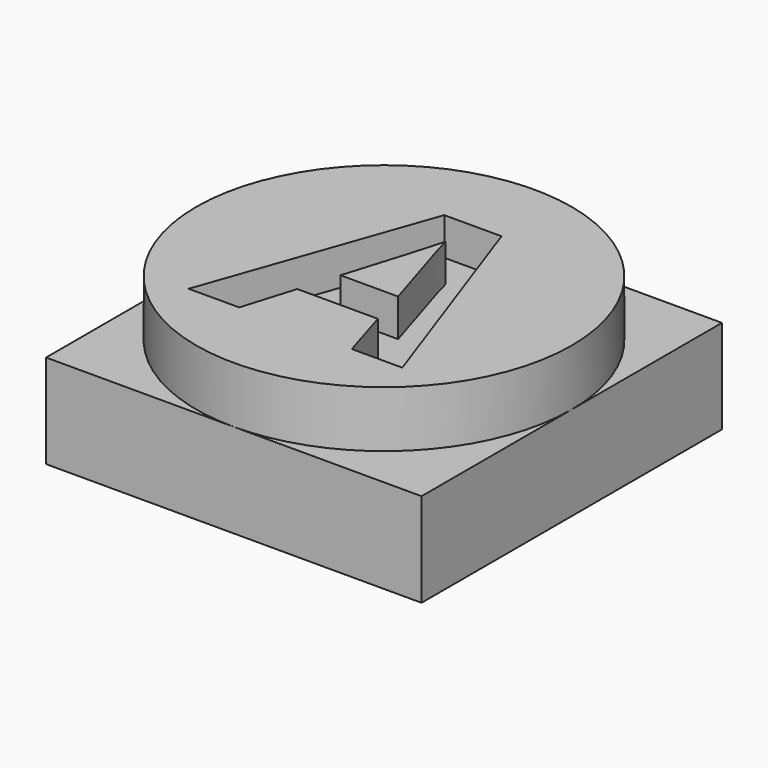
from build123d import *

# Parameters (mm, degrees)
F0_W         = 20
F0_H         = 20
F1_DEPTH     = 5
F2_R         = 10
F3_DEPTH     = 3
F4_TEXT_SIZE = 16.4918847279
F5_DEPTH     = 2


# Not quite as in the source:
# - Text() gives the source's letters only with a copy of the font that has no kerning and outlines rounded to 1/6400 em; it was checked with that copy


with BuildPart() as f1:
    # F0 (on Top) → F1 (new body)
    with BuildSketch(Plane.XY):
        Rectangle(F0_W, F0_H)
    extrude(amount=F1_DEPTH)

    # F2 (on face) → F3 (join)
    with BuildSketch(Plane.XY.offset(5)):
        Circle(F2_R)
    extrude(amount=F3_DEPTH)

    # F4 (on face) → F5 (cut)
    with BuildSketch(Plane.XY.offset(8)):
        with Locations((-5.636760965, -5.9601804242)):
            Text('A', F4_TEXT_SIZE, font='Open Sans', font_style=FontStyle.BOLD, text_align=(TextAlign.LEFT, TextAlign.BOTTOM))
    extrude(amount=-F5_DEPTH, mode=Mode.SUBTRACT)


solid = f1.part
